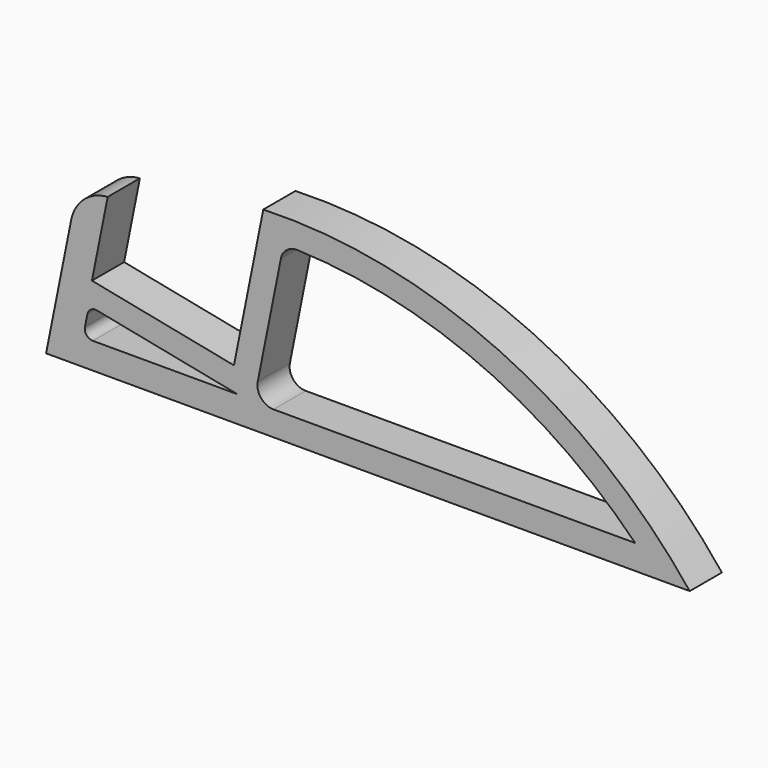
from build123d import *

# Parameters (mm, degrees)
F1_DEPTH    = 76.2
F2_R        = 2.54
F3_R        = 1.27
F4_T1_DEPTH = 102.1482316142
F5_DEPTH    = 69.85


# Not quite as in the source:
# - a fillet or chamfer that OpenCascade refuses, or shapes differently, is made with other operations: its cross-section is extruded or revolved along the edge and cut away or added


with BuildPart() as f1:
    # F0 (on Front) → F1 (new body)
    with BuildSketch(Plane.XZ):
        with BuildLine():
            Line((-38.6677846295, 20.0523413639), (-43.4175846295, 20.0523413639))
            Line((-43.4175846295, 20.0523413639), (-48.3946166933, -4.8552709632))
            Line((-48.3946166933, -4.8552709632), (53.2053833067, -4.8552709632))
            ThreePointArc((53.2053833067, -4.8552709632), (23.2548005589, 18.7290020933), (-14.1116172914, 26.2792444457))
            Line((-14.1116172914, 26.2792444457), (-18.739449567, 3.119206343))
            Line((-18.739449567, 3.119206343), (-41.1563006614, 7.5985352004))
            Line((-41.1563006614, 7.5985352004), (-38.6677846295, 20.0523413639))
        make_face()
        Polygon((-41.6217533096, 3.9728981134), (-18.1607622718, -0.7150704927), (-42.558501873, -0.7150704927), align=None, mode=Mode.SUBTRACT)
        with BuildLine():
            ThreePointArc((-10.9155429452, 22.4410306257), (19.1784355797, 16.2823947845), (44.5942434068, -0.9690704107))
            Line((44.5942434068, -0.9690704107), (-15.5933427256, -0.9690704107))
            Line((-15.5933427256, -0.9690704107), (-10.9155429452, 22.4410306257))
        make_face(mode=Mode.SUBTRACT)
    extrude(amount=F1_DEPTH)

    # F2
    f2_edges = [f1.edges().sort_by_distance(p)[0] for p in [
        (-10.915543, -38.1, 22.441031),
        (-15.593343, -38.1, -0.96907),
    ]]
    fillet(f2_edges, radius=F2_R)

    # F3
    f3_edges = [f1.edges().sort_by_distance(p)[0] for p in [
        (-41.621753, -38.1, 3.972898),
        (-42.558502, -38.1, -0.71507),
    ]]
    fillet(f3_edges, radius=F3_R)

    # F4: fillet of radius 6.35 on 1 edges, made by hand

    # F4_s2 → F4_t1 (cut)
    with BuildSketch(Plane.XZ.offset(-12.9741158071)):
        with BuildLine():
            ThreePointArc((-38.6677846295, 20.0523413639), (-42.4092351432, 18.4801883775), (-44.4344758164, 14.9632981071))
            Line((-44.4344758164, 14.9632981071), (-43.4175846295, 20.0523413639))
            Line((-43.4175846295, 20.0523413639), (-38.6677846295, 20.0523413639))
        make_face()
    extrude(amount=F4_T1_DEPTH, mode=Mode.SUBTRACT)

    # F5 (cut): a face of the model
    f5_faces = [f1.faces().sort_by_distance(p)[0] for p in [
        (-45.3723710361, -76.2, 4.845766414),
    ]]
    extrude(f5_faces, amount=-F5_DEPTH, mode=Mode.SUBTRACT)


solid = f1.part
